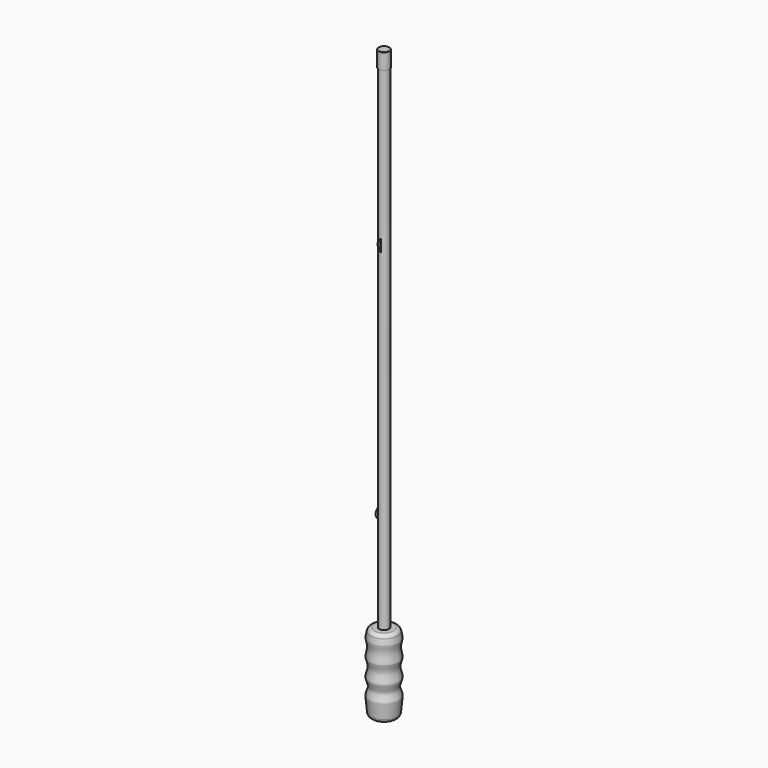
from build123d import *

# Parameters (mm, degrees)
F2_R      = 7.9375
F3_DEPTH  = 892.175
F5_DEPTH  = 0.79375
F7_DEPTH  = 1.5875
F8_R      = 8.7071969697
F8_R_2    = 7.9375
F9_DEPTH  = 0.7696969697
F10_DEPTH = 25.4
F11_R     = 0.769687


# Not quite as in the source:
# - a fillet or chamfer is up to 0.001 mm smaller than in the source, because OpenCascade refuses the exact size


with BuildPart() as f1:
    # F0 (on Front) → F1 (revolve)
    with BuildSketch(Plane.XZ):
        with BuildLine():
            Line((15.7668136708, 65.9038792952), (0, 66.1711168233))
            Line((0, 66.1711168233), (0, -60.618262738))
            Line((0, -60.618262738), (15.24, -60.618262738))
            ThreePointArc((15.24, -60.618262738), (19.5776834861, -58.9058269666), (21.5758380378, -54.6921216277))
            add(Edge.make_bspline(
                [(21.5758380378, -54.6921216277), (22.0121080476, -48.1707623027), (23.5004956481, -33.7347059012), (24.3273034079, -29.2104516541), (18.1620396435, -18.1540798034), (24.0703888205, -6.9294910192), (23.8921343024, -1.879261787), (18.6881535155, 10.0722464342), (23.9231717284, 22.4458200693), (23.6328702389, 26.0908705285), (20.3031790042, 38.9499451611), (23.7086494403, 49.9464189693), (23.7712381176, 52.9070726894), (22.4122901354, 58.0076061581), (21.8994664046, 60.7301988849)],
                knots=[0.0355569573, 0.0355569573, 0.0355569573, 0.0355569573, 0.1339530606, 0.1992024509, 0.2872295991, 0.3775566826, 0.4359175184, 0.5293405972, 0.6227636718, 0.6733056322, 0.7683398311, 0.8564828563, 0.9070248167, 0.9634390062, 0.9634390062, 0.9634390062, 0.9634390062], degree=3))
            ThreePointArc((21.8994664046, 60.7301988849), (19.7537865223, 64.4083328563), (15.7668136708, 65.9038792952))
        make_face()
    revolve(axis=Axis((0, 0, 2.7764270426), (0, 0, -1)))

    # F2 (on Top) → F3 (join)
    with BuildSketch(Plane.XY):
        Circle(F2_R)
    extrude(amount=F3_DEPTH)


with BuildPart() as f5:
    # F4 (on Front) → F5 (new body, symmetric)
    with BuildSketch(Plane.XZ):
        with BuildLine():
            Line((-7.9375, 218.5711168233), (-5.3975, 218.5711168233))
            Line((-5.3975, 218.5711168233), (-5.3975, 237.6211168233))
            Line((-5.3975, 237.6211168233), (-7.9375, 237.6211168233))
            add(Edge.make_bspline(
                [(-11.1125, 218.5711168233), (-16.0493329167, 224.8954027891), (-10.2215753868, 233.1035137177), (-7.9375, 237.6211168233)],
                knots=[0, 0, 0, 0, 19.3127710337, 19.3127710337, 19.3127710337, 19.3127710337], degree=3))
            Line((-11.1125, 218.5711168233), (-7.9375, 218.5711168233))
        make_face()
    extrude(amount=F5_DEPTH, both=True)


with BuildPart() as f7:
    # F6 (on Right) → F7 (new body)
    with BuildSketch(Plane.YZ):
        with BuildLine():
            Line((-5.3975, 605.79), (-5.3975, 624.84))
            Line((-5.3975, 624.84), (-7.9375, 624.84))
            Line((-7.9375, 624.84), (-11.1125, 624.84))
            add(Edge.make_bspline(
                [(-11.1125, 624.84), (-16.0493329167, 618.5157140341), (-10.2215753868, 610.3076031056), (-7.9375, 605.79)],
                knots=[0, 0, 0, 0, 19.3127710337, 19.3127710337, 19.3127710337, 19.3127710337], degree=3))
            Line((-7.9375, 605.79), (-5.3975, 605.79))
        make_face()
    extrude(amount=F7_DEPTH)


with BuildPart() as f9:
    # F8 (on face) → F9 (new body)
    with BuildSketch(Plane.XY.offset(892.175)):
        Circle(F8_R)
        Circle(F8_R_2, mode=Mode.SUBTRACT)
        Circle(F8_R_2)
    extrude(amount=F9_DEPTH)

    # F8 (on face) → F10 (join)
    with BuildSketch(Plane.XY.offset(892.175)):
        Circle(F8_R)
        Circle(F8_R_2, mode=Mode.SUBTRACT)
    extrude(amount=-F10_DEPTH)

    # F11 (radius 0.7696969697 in the source; OpenCascade refuses exactly that, so slightly less here)
    f11_edges = [f9.edges().sort_by_distance(p)[0] for p in [
        (-8.707197, 0, 892.944697),
    ]]
    fillet(f11_edges, radius=F11_R)


solid = Compound([f1.part, f5.part, f7.part, f9.part])
